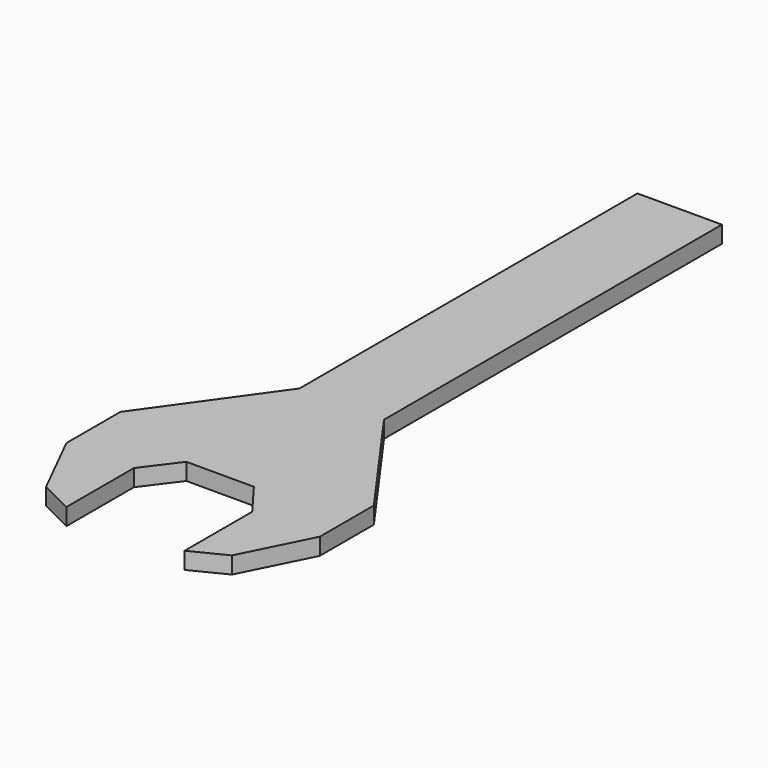
from build123d import *

# Parameters (mm, degrees)
F1_DEPTH = 10


# Not quite as in the source:
# - a feature of the source that left no trace in its solid (it failed there, or was rolled back) is left out


with BuildPart() as f1:
    # F0 (on Top) → F1 (new body)
    with BuildSketch(Plane.XY):
        Polygon((-35, -20), (-20, 0), (20, 0), (35, -20), (35, -70), (55, -60), (75, -20), (75, 20), (25, 90), (25, 340), (-25, 340), (-25, 90), (-75, 20), (-75, -20), (-55, -60), (-35, -70), align=None)
    extrude(amount=F1_DEPTH)


solid = f1.part
